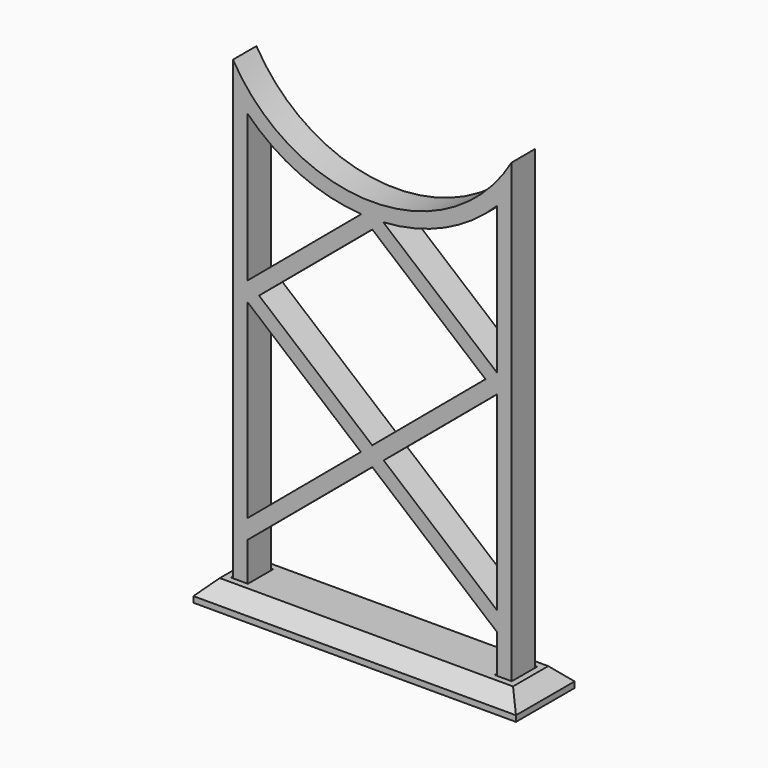
from build123d import *

# Parameters (mm, degrees)
F0_W          = 120.65
F0_H          = 12.7
F1_DEPTH      = 228.6
F3_DEPTH      = 25.4
F3_DEPTH_BACK = 25.4
F4_W          = 139.7
F4_H          = 31.75
F4_W_2        = 7.366
F4_H_2        = 13.716
F5_DEPTH      = 6.35
F6_SIZE       = 6.34999
F7_DEPTH      = 2.54


# Not quite as in the source:
# - a fillet or chamfer is up to 0.001 mm smaller than in the source, because OpenCascade refuses the exact size


with BuildPart() as f1:
    # F0 (on Top) → F1 (new body)
    with BuildSketch(Plane.XY):
        Rectangle(F0_W, F0_H)
    extrude(amount=F1_DEPTH)

    # F2 (on Front) → F3 (cut, two sides)
    with BuildSketch(Plane.XZ) as f3_sk:
        with BuildLine():
            ThreePointArc((60.325, 203.7592132588), (67.4267148466, 220.7326802639), (69.85, 238.9716666667))
            ThreePointArc((69.85, 238.9716666667), (-18.2389864028, 306.3983815132), (-60.325, 203.7592132588))
            ThreePointArc((-60.325, 203.7592132588), (0, 169.1216666667), (60.325, 203.7592132588))
        make_face()
        with BuildLine():
            ThreePointArc((-4.7619259855, 162.9206044722), (-31.407301592, 169.5452926672), (-53.975, 185.1837556178))
            Line((-53.975, 185.1837556178), (-53.975, 121.6259322175))
            Line((-53.975, 121.6259322175), (-4.7619259855, 162.9206044722))
        make_face()
        with BuildLine():
            Line((53.975, 121.6259322175), (53.975, 185.1837556178))
            ThreePointArc((53.975, 185.1837556178), (31.407301592, 169.5452926672), (4.7619259855, 162.9206044722))
            Line((4.7619259855, 162.9206044722), (53.975, 121.6259322175))
        make_face()
        Polygon((0, 158.626998523), (-49.0355768497, 117.4812640739), (0, 76.3355296247), (49.0355768497, 117.4812640739), align=None)
        Polygon((-4.9394231503, 72.1908614811), (-53.975, 113.3365959302), (-53.975, 31.0451270319), align=None)
        Polygon((53.975, 31.0451270319), (53.975, 113.3365959302), (4.9394231503, 72.1908614811), align=None)
        Polygon((-53.975, 22.7557907447), (-53.975, 0), (53.975, 0), (53.975, 22.7557907447), (0, 68.0461933374), align=None)
    extrude(amount=-F3_DEPTH, mode=Mode.SUBTRACT)
    extrude(f3_sk.sketch, amount=F3_DEPTH_BACK, mode=Mode.SUBTRACT)


with BuildPart() as f5:
    # F4 (on Top) → F5 (new body)
    with BuildSketch(Plane.XY):
        Rectangle(F4_W, F4_H)
        with Locations((-57.15, 0)):
            Rectangle(F4_W_2, F4_H_2, mode=Mode.SUBTRACT)
        with Locations((57.15, 0)):
            Rectangle(F4_W_2, F4_H_2, mode=Mode.SUBTRACT)
    extrude(amount=F5_DEPTH)

    # F6 (size 6.35 in the source; OpenCascade refuses exactly that, so slightly less here)
    f6_edges = [f5.edges().sort_by_distance(p)[0] for p in [
        (0, -15.875, 6.35),
        (-69.85, 0, 6.35),
        (0, 15.875, 6.35),
        (69.85, 0, 6.35),
    ]]
    chamfer(f6_edges, length=F6_SIZE)

    # F4 (on Top) → F7 (join)
    with BuildSketch(Plane.XY):
        Rectangle(F4_W, F4_H)
        with Locations((-57.15, 0)):
            Rectangle(F4_W_2, F4_H_2, mode=Mode.SUBTRACT)
        with Locations((57.15, 0)):
            Rectangle(F4_W_2, F4_H_2, mode=Mode.SUBTRACT)
        with Locations((-57.15, 0)):
            Rectangle(F4_W_2, F4_H_2)
        with Locations((57.15, 0)):
            Rectangle(F4_W_2, F4_H_2)
    extrude(amount=-F7_DEPTH)


solid = Compound([f1.part, f5.part])
